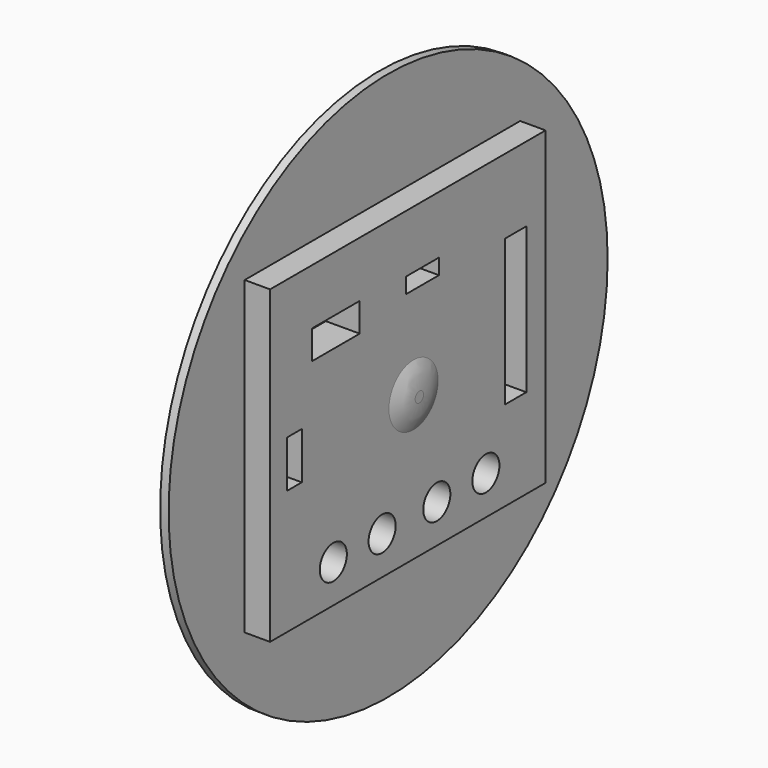
from build123d import *

# Parameters (mm, degrees)
F0_W      = 51.6687010021
F0_H      = 46.5666760604
F0_R      = 2.54
F0_W_2    = 2.7420800179
F0_H_2    = 7.0510646328
F0_W_3    = 8.9598344539
F0_H_3    = 4.3325314605
F0_R_2    = 4.6152632683
F0_W_4    = 4.0421821177
F0_H_4    = 21.9193678349
F0_W_5    = 6.2187388539
F0_H_5    = 2.331847325
F7_DEPTH  = 5.08
F8_DEPTH  = 5.95595
F0_R_3    = 41.1742131812
F10_DEPTH = 1.27


# Not quite as in the source:
# - a fillet or chamfer that OpenCascade refuses, or shapes differently, is made with other operations: its cross-section is extruded or revolved along the edge and cut away or added
# - the program builds the solid bodies; features that only make, move or delete a surface that nothing else refers to are left out


with BuildPart() as f7:
    # F0 (on Right) → F7 (new body)
    with BuildSketch(Plane.YZ):
        with Locations((-1.069343959, 1.5875007549)):
            Rectangle(F0_W, F0_H)
        with Locations((-15.0437285019, -15.973794371)):
            Circle(F0_R, mode=Mode.SUBTRACT)
        with Locations((-5.8897222223, -15.9437051803)):
            Circle(F0_R, mode=Mode.SUBTRACT)
        with Locations((4.3680206165, -15.9099880108)):
            Circle(F0_R, mode=Mode.SUBTRACT)
        with Locations((13.5722881269, -15.8797336116)):
            Circle(F0_R, mode=Mode.SUBTRACT)
        with Locations((-22.3283721134, 0.4896570463)):
            Rectangle(F0_W_2, F0_H_2, mode=Mode.SUBTRACT)
        with Locations((-14.5700857925, 14.3513671276)):
            Rectangle(F0_W_3, F0_H_3, mode=Mode.SUBTRACT)
        Circle(F0_R_2, mode=Mode.SUBTRACT)
        with Locations((19.1379059106, 2.7070390061)):
            Rectangle(F0_W_4, F0_H_4, mode=Mode.SUBTRACT)
        with Locations((1.6578678042, 15.0334504433)):
            Rectangle(F0_W_5, F0_H_5, mode=Mode.SUBTRACT)
    extrude(amount=F7_DEPTH)

    # F0 (on Right) → F8 (join)
    with BuildSketch(Plane.YZ):
        Circle(F0_R_2)
    extrude(amount=F8_DEPTH)

    # F9: fillet of radius 8.7940626066 on 1 edges, made by hand

    # F9_s1 → F9_t2 (revolve, cut)
    with BuildSketch(Plane.XY):
        with BuildLine():
            ThreePointArc((5.08, 4.6152632683), (5.7341658279, 2.7517089067), (5.95595, 0.7891647492))
            Line((5.95595, 0.7891647492), (5.95595, 4.6152632683))
            Line((5.95595, 4.6152632683), (5.08, 4.6152632683))
        make_face()
    revolve(axis=Axis((5.95595, 0, 0), (1, 0, 0)), mode=Mode.SUBTRACT)


with BuildPart() as f10:
    # F0 (on Right) → F10 (new body)
    with BuildSketch(Plane.YZ):
        Circle(F0_R_3)
        with Locations((-1.069343959, 1.5875007549)):
            Rectangle(F0_W, F0_H, mode=Mode.SUBTRACT)
    extrude(amount=F10_DEPTH)


solid = Compound([f7.part, f10.part])
